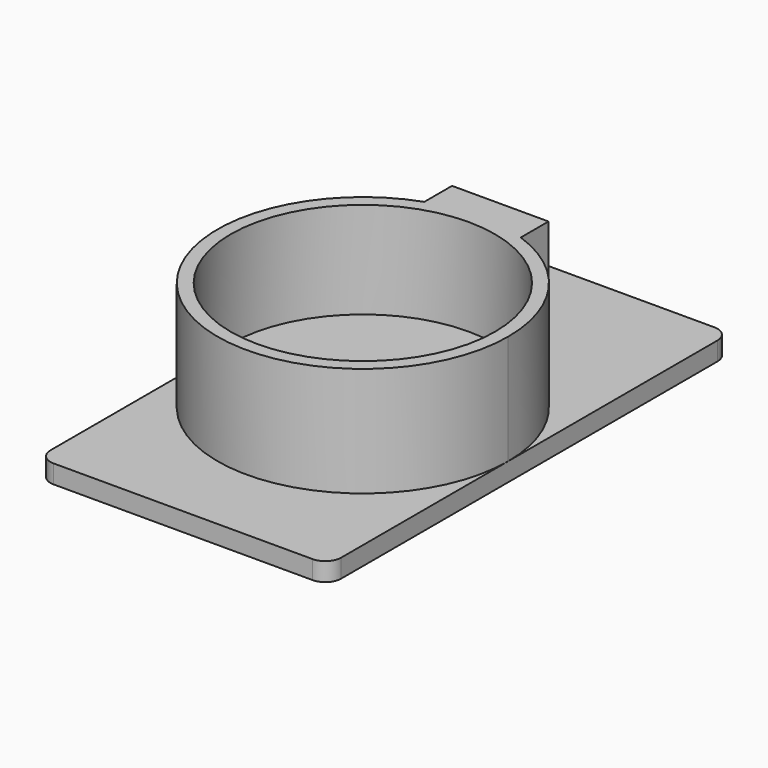
from build123d import *

# Parameters (mm, degrees)
F0_W     = 22
F0_H     = 38
F1_DEPTH = 1.4
F2_R     = 1.2
F3_R     = 10
F4_DEPTH = 8.3
F5_DEPTH = 1


with BuildPart() as f1:
    # F0 (on Top) → F1 (new body)
    with BuildSketch(Plane.XY):
        Rectangle(F0_W, F0_H)
    extrude(amount=F1_DEPTH)

    # F2
    f2_edges = [f1.edges().sort_by_distance(p)[0] for p in [
        (-11, 19, 0.7),
        (11, 19, 0.7),
        (-11, -19, 0.7),
        (11, -19, 0.7),
    ]]
    fillet(f2_edges, radius=F2_R)


with BuildPart() as f4:
    # F3 (on face) → F4 (new body)
    with BuildSketch(Plane.XY.offset(1.4)):
        with BuildLine():
            ThreePointArc((-3.65, 8.3767769563), (-6.3580657436, -10.976357836), (11, -2))
            ThreePointArc((11, -2), (8.976357836, 4.3580657436), (3.65, 8.3767769563))
            Line((3.65, 8.3767769563), (-3.65, 8.3767769563))
        make_face()
        with Locations((0, -2)):
            Circle(F3_R, mode=Mode.SUBTRACT)
        with BuildLine():
            Line((-3.65, 8.3767769563), (3.65, 8.3767769563))
            ThreePointArc((3.65, 8.3767769563), (0, 9), (-3.65, 8.3767769563))
        make_face()
        with BuildLine():
            ThreePointArc((-3.65, 8.3767769563), (0, 9), (3.65, 8.3767769563))
            Line((3.65, 8.3767769563), (3.65, 11))
            Line((3.65, 11), (-3.65, 11))
            Line((-3.65, 11), (-3.65, 8.3767769563))
        make_face()
    extrude(amount=F4_DEPTH)

    # F3 (on face) → F5 (join)
    with BuildSketch(Plane.XY.offset(1.4)):
        with Locations((0, -2)):
            Circle(F3_R)
    extrude(amount=F5_DEPTH)


solid = Compound([f1.part, f4.part])
